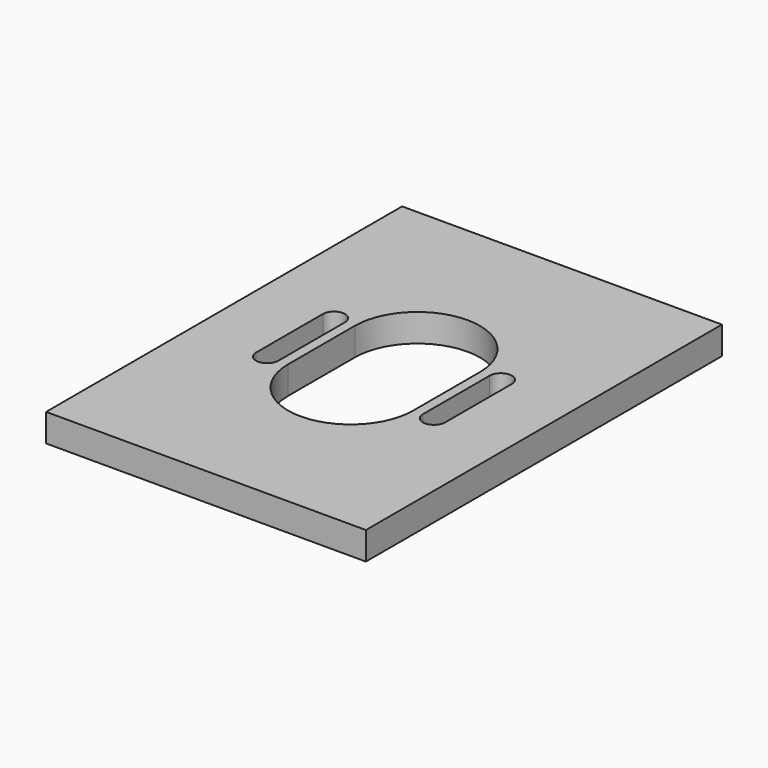
from build123d import *

# Parameters (mm, degrees)
F0_W     = 115
F0_H     = 160
F1_DEPTH = 10
F3_DEPTH = 10.001


# Not quite as in the source:
# - a pattern or mirror of a feature is missing from the dataset's text; its kind, count and spacing are read off the source's solid


with BuildPart() as f1:
    # F0 (on Top) → F1 (new body)
    with BuildSketch(Plane.XY):
        Rectangle(F0_W, F0_H)
        with BuildLine():
            Line((-22.5, -15), (-22.5, 15))
            ThreePointArc((-22.5, 15), (0, 37.5), (22.5, 15))
            Line((22.5, 15), (22.5, -15))
            ThreePointArc((22.5, -15), (0, -37.5), (-22.5, -15))
        make_face(mode=Mode.SUBTRACT)
    extrude(amount=F1_DEPTH)

    # F2 (on face) → F3 (cut, through all)
    with BuildSketch(Plane.XY.offset(10)):
        with BuildLine():
            ThreePointArc((-26, 15), (-30, 19), (-34, 15))
            Line((-34, 15), (-34, -15))
            ThreePointArc((-34, -15), (-30, -19), (-26, -15))
            Line((-26, -15), (-26, 0))
            Line((-26, 0), (-26, 15))
        make_face()
    f3 = extrude(amount=-F3_DEPTH, mode=Mode.SUBTRACT)

    # F3_copies: F3 across plane
    add(f3.mirror(Plane(origin=(0, 0, 0), x_dir=(0, 0, 1), z_dir=(1, 0, 0))), mode=Mode.SUBTRACT)


solid = f1.part
